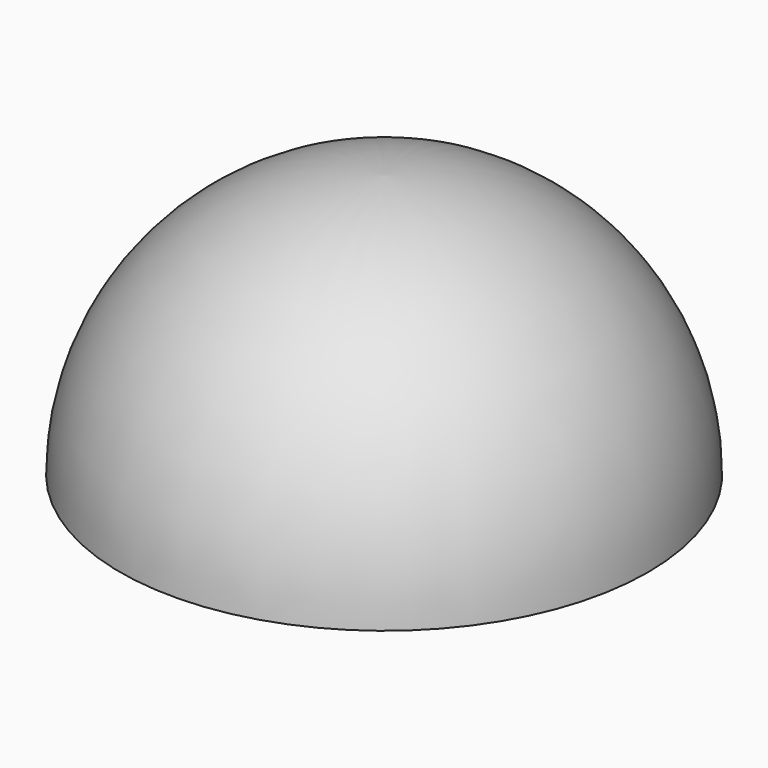
from build123d import *

# Parameters (mm, degrees)
F0_R     = 5.003047497
F1_DEPTH = 5
F2_R     = 4.99999


# Not quite as in the source:
# - a fillet or chamfer is up to 0.001 mm smaller than in the source, because OpenCascade refuses the exact size


with BuildPart() as f1:
    # F0 (on Top) → F1 (new body)
    with BuildSketch(Plane.XY):
        with Locations((-8.2363244146, 7.1773678064)):
            Circle(F0_R)
    extrude(amount=F1_DEPTH)

    # F2 (radius 5 in the source; OpenCascade refuses exactly that, so slightly less here)
    f2_edges = [f1.edges().sort_by_distance(p)[0] for p in [
        (-13.239372, 7.177368, 5),
    ]]
    fillet(f2_edges, radius=F2_R)


solid = f1.part
